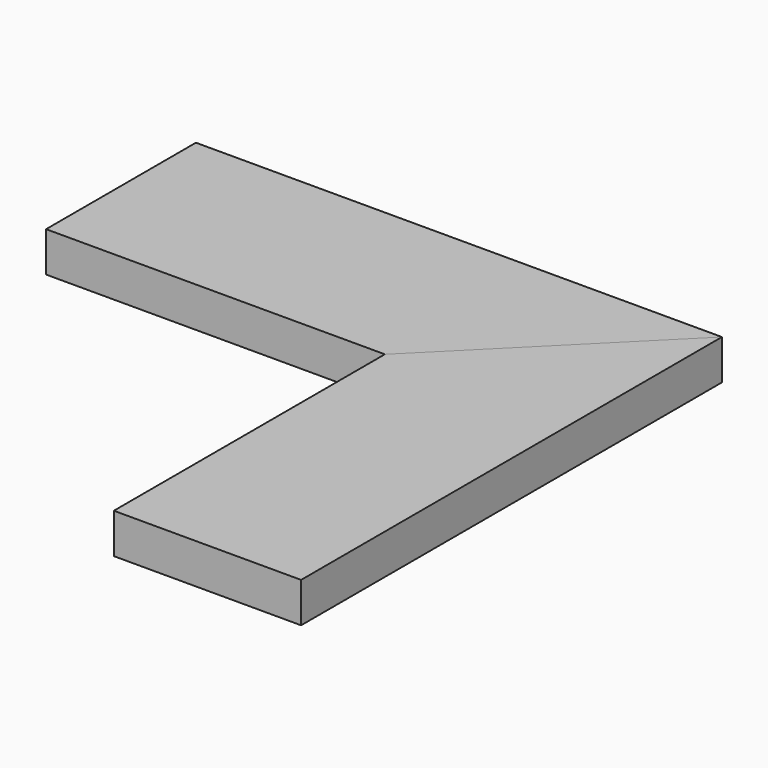
from build123d import *

# Parameters (mm, degrees)
F0_W     = 250
F0_H     = 89
F1_DEPTH = 19
F2_W     = 89
F2_H     = 250
F3_DEPTH = 19
F5_DEPTH = 19.001
F7_DEPTH = 9.5


with BuildPart() as f1:
    # F0 (on Top) → F1 (new body)
    with BuildSketch(Plane.XY):
        with Locations((-125, -44.5)):
            Rectangle(F0_W, F0_H)
    extrude(amount=F1_DEPTH)

    # F4 (on face) → F5 (cut, through all)
    with BuildSketch(Plane.XY.offset(19)):
        Polygon((0, -89), (0, 0), (-89, -89), align=None)
    extrude(amount=-F5_DEPTH, mode=Mode.SUBTRACT)

    # F6 (on face) → F7 (cut)
    with BuildSketch(Plane(origin=(0, 0, 0), x_dir=(1, 0, 0), z_dir=(0, 0, -1))):
        Polygon((0, 0), (-89, 89), (-89, 0), align=None)
    extrude(amount=-F7_DEPTH, mode=Mode.SUBTRACT)


with BuildPart() as f3:
    # F2 (on Top) → F3 (new body)
    with BuildSketch(Plane.XY):
        with Locations((-44.5, -125)):
            Rectangle(F2_W, F2_H)
    extrude(amount=F3_DEPTH)

    # F8: cut F1
    add(f1.part, mode=Mode.SUBTRACT)


solid = Compound([f1.part, f3.part])
